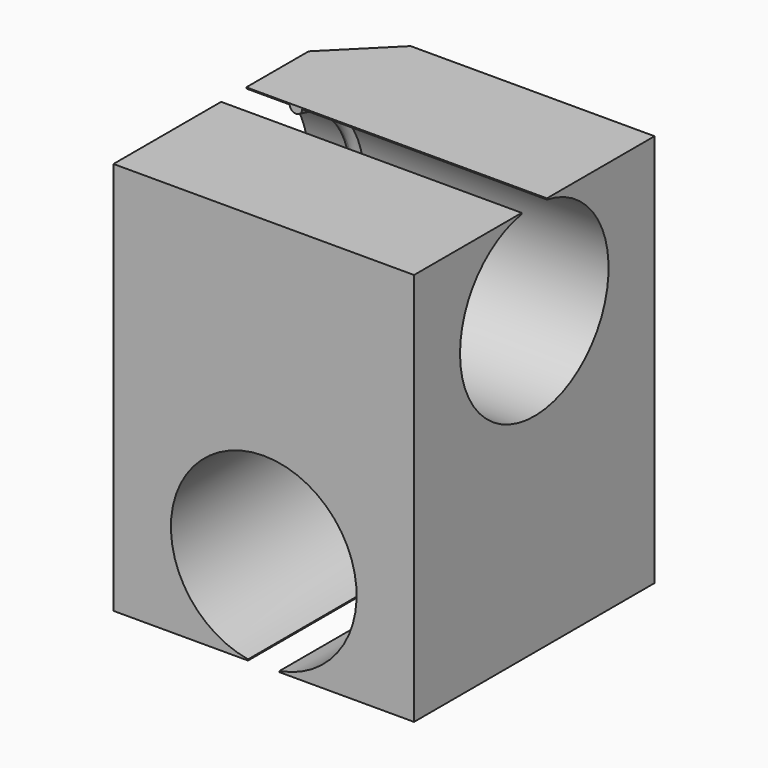
from build123d import *

# Parameters (mm, degrees)
F0_W          = 24.257
F0_H          = 24.257
F1_DEPTH      = 31.75
F3_DEPTH      = 25.4
F5_DEPTH      = 25.4
F9_DEPTH      = 1.016
F11_DEPTH     = 1.016
F12_T4_ANGLE  = 359.64
F12_S5_R      = 7.493
F12_T6_DEPTH  = 13
F12_T10_ANGLE = 359.64
F12_S11_R     = 7.493
F12_T12_DEPTH = 13
F12_T16_ANGLE = 359.64
F12_S17_R     = 7.493
F12_T18_DEPTH = 14
F12_T22_ANGLE = 359.64
F12_S23_R     = 7.493
F12_T24_DEPTH = 14
F13_SIZE      = 4.572


# Not quite as in the source:
# - a fillet or chamfer that OpenCascade refuses, or shapes differently, is made with other operations: its cross-section is extruded or revolved along the edge and cut away or added


with BuildPart() as f1:
    # F0 (on Top) → F1 (new body)
    with BuildSketch(Plane.XY):
        Rectangle(F0_W, F0_H)
    extrude(amount=F1_DEPTH)

    # F2 (on face) → F3 (cut)
    with BuildSketch(Plane.XZ.offset(12.1285)):
        with BuildLine():
            Line((1.27, 0), (1.27, 0.0893613859))
            ThreePointArc((1.27, 0.0893613859), (0, 14.96695), (-1.27, 0.0893613859))
            Line((-1.27, 0.0893613859), (-1.27, 0))
            Line((-1.27, 0), (1.27, 0))
        make_face()
    extrude(amount=-F3_DEPTH, mode=Mode.SUBTRACT)

    # F4 (on face) → F5 (cut)
    with BuildSketch(Plane(origin=(-12.1285, 0, 0), x_dir=(0, -1, 0), z_dir=(-1, 0, 0))):
        with BuildLine():
            ThreePointArc((-1.27, 31.6606386141), (-4.8285059283, 18.5462524905), (7.493, 24.27605))
            ThreePointArc((7.493, 24.27605), (5.7297975095, 29.1045559283), (1.27, 31.6606386141))
            ThreePointArc((1.27, 31.6606386141), (0.9030893061, 31.7144287686), (0.5339666633, 31.75))
            Line((0.5339666633, 31.75), (-0.5339666633, 31.75))
            ThreePointArc((-0.5339666633, 31.75), (-0.9030893061, 31.7144287686), (-1.27, 31.6606386141))
        make_face()
        with BuildLine():
            ThreePointArc((0.5339666633, 31.75), (0.9030893061, 31.7144287686), (1.27, 31.6606386141))
            Line((1.27, 31.6606386141), (1.27, 31.75))
            Line((1.27, 31.75), (0.5339666633, 31.75))
        make_face()
        with BuildLine():
            Line((-1.27, 31.75), (-1.27, 31.6606386141))
            ThreePointArc((-1.27, 31.6606386141), (-0.9030893061, 31.7144287686), (-0.5339666633, 31.75))
            Line((-0.5339666633, 31.75), (-1.27, 31.75))
        make_face()
        with BuildLine():
            Line((-0.5339666633, 31.75), (0.5339666633, 31.75))
            ThreePointArc((0.5339666633, 31.75), (0, 31.76905), (-0.5339666633, 31.75))
        make_face()
    extrude(amount=-F5_DEPTH, mode=Mode.SUBTRACT)

    # F8 (on offset) → F9 (join)
    with BuildSketch(Plane(origin=(-8.62838, 0, 0), x_dir=(0, -1, 0), z_dir=(-1, 0, 0))):
        with BuildLine():
            Line((-1.27, 31.1704541193), (-1.27, 31.6606386141))
            ThreePointArc((-1.27, 31.6606386141), (0, 16.78305), (1.27, 31.6606386141))
            Line((1.27, 31.6606386141), (1.27, 31.1704541193))
            ThreePointArc((1.27, 31.1704541193), (0, 17.26565), (-1.27, 31.1704541193))
        make_face()
    extrude(amount=-F9_DEPTH)

    # F10 (on offset) → F11 (join)
    with BuildSketch(Plane(origin=(0, 8.62838, 0), x_dir=(-1, 0, 0), z_dir=(0, 1, 0))):
        with BuildLine():
            ThreePointArc((1.27, 0.0893613859), (0, 14.96695), (-1.27, 0.0893613859))
            Line((-1.27, 0.0893613859), (-1.27, 0.5795458807))
            ThreePointArc((-1.27, 0.5795458807), (0, 14.48435), (1.27, 0.5795458807))
            Line((1.27, 0.5795458807), (1.27, 0.0893613859))
        make_face()
    extrude(amount=-F11_DEPTH)

    # F12: fillet of radius 0.508 on 4 edges, made by hand


with BuildPart() as f12_tool2:
    # F12_s3 → F12_t4 (revolve)
    with BuildSketch(Plane(origin=(0.0234799519, 0, 7.37647e-05), x_dir=(0, 1, 0), z_dir=(-0.9999950652, 0, -0.0031415875))):
        with BuildLine():
            ThreePointArc((8.62838, 0.0444868824), (8.4795902448, -0.3147233624), (8.12038, -0.4635131176))
            Line((8.12038, -0.4635131176), (8.62838, -0.4635131176))
            Line((8.62838, -0.4635131176), (8.62838, 0.0444868824))
        make_face()
    revolve(axis=Axis((0, 8.62838, 7.47395), (0, -1, 0)), revolution_arc=F12_T4_ANGLE)

    # F12_s5 → F12_t6 (intersect, symmetric)
    with BuildSketch(Plane.XZ.offset(-8.2)):
        with Locations((0, 7.47395)):
            Circle(F12_S5_R)
    extrude(amount=F12_T6_DEPTH, both=True, mode=Mode.INTERSECT)


with BuildPart() as f1_1:
    add(f1.part)

    # F12_t1: cut F12_tool2
    add(f12_tool2.part, mode=Mode.SUBTRACT)


with BuildPart() as f12_tool8:
    # F12_s9 → F12_t10 (revolve)
    with BuildSketch(Plane(origin=(0.0234799519, 0, 7.37647e-05), x_dir=(0, 1, 0), z_dir=(-0.9999950652, 0, -0.0031415875))):
        with BuildLine():
            ThreePointArc((7.61238, 0.0444868824), (7.7611697552, -0.3147233624), (8.12038, -0.4635131176))
            Line((8.12038, -0.4635131176), (7.61238, -0.4635131176))
            Line((7.61238, -0.4635131176), (7.61238, 0.0444868824))
        make_face()
    revolve(axis=Axis((0, 7.61238, 7.47395), (0, -1, 0)), revolution_arc=F12_T10_ANGLE)

    # F12_s11 → F12_t12 (intersect, symmetric)
    with BuildSketch(Plane.XZ.offset(-7.9)):
        with Locations((0, 7.47395)):
            Circle(F12_S11_R)
    extrude(amount=F12_T12_DEPTH, both=True, mode=Mode.INTERSECT)


with BuildPart() as f1_2:
    add(f1_1.part)

    # F12_t7: cut F12_tool8
    add(f12_tool8.part, mode=Mode.SUBTRACT)


with BuildPart() as f12_tool14:
    # F12_s15 → F12_t16 (revolve)
    with BuildSketch(Plane(origin=(0, 0.0762649585, 0.0002395942), x_dir=(1, 0, 0), z_dir=(0, 0.9999950652, 0.0031415875))):
        with BuildLine():
            ThreePointArc((-7.61238, -31.7943302026), (-7.7611697552, -31.4351199578), (-8.12038, -31.2863302026))
            Line((-8.12038, -31.2863302026), (-7.61238, -31.2863302026))
            Line((-7.61238, -31.2863302026), (-7.61238, -31.7943302026))
        make_face()
    revolve(axis=Axis((-7.61238, 0, 24.27605), (1, 0, 0)), revolution_arc=F12_T16_ANGLE)

    # F12_s17 → F12_t18 (intersect, symmetric)
    with BuildSketch(Plane.YZ.offset(-8)):
        with Locations((0, 24.27605)):
            Circle(F12_S17_R)
    extrude(amount=F12_T18_DEPTH, both=True, mode=Mode.INTERSECT)


with BuildPart() as f1_3:
    add(f1_2.part)

    # F12_t13: cut F12_tool14
    add(f12_tool14.part, mode=Mode.SUBTRACT)


with BuildPart() as f12_tool20:
    # F12_s21 → F12_t22 (revolve)
    with BuildSketch(Plane(origin=(0, 0.0762649585, 0.0002395942), x_dir=(1, 0, 0), z_dir=(0, 0.9999950652, 0.0031415875))):
        with BuildLine():
            ThreePointArc((-8.12038, -31.2863302026), (-8.4795902448, -31.4351199578), (-8.62838, -31.7943302026))
            Line((-8.62838, -31.7943302026), (-8.62838, -31.2863302026))
            Line((-8.62838, -31.2863302026), (-8.12038, -31.2863302026))
        make_face()
    revolve(axis=Axis((-8.62838, 0, 24.27605), (1, 0, 0)), revolution_arc=F12_T22_ANGLE)

    # F12_s23 → F12_t24 (intersect, symmetric)
    with BuildSketch(Plane.YZ.offset(-8.4)):
        with Locations((0, 24.27605)):
            Circle(F12_S23_R)
    extrude(amount=F12_T24_DEPTH, both=True, mode=Mode.INTERSECT)


with BuildPart() as f1_4:
    add(f1_3.part)

    # F12_t19: cut F12_tool20
    add(f12_tool20.part, mode=Mode.SUBTRACT)

    # F13
    f13_edges = [f1_4.edges().sort_by_distance(p)[0] for p in [
        (-12.1285, 12.1285, 15.875),
    ]]
    chamfer(f13_edges, length=F13_SIZE)


solid = f1_4.part
